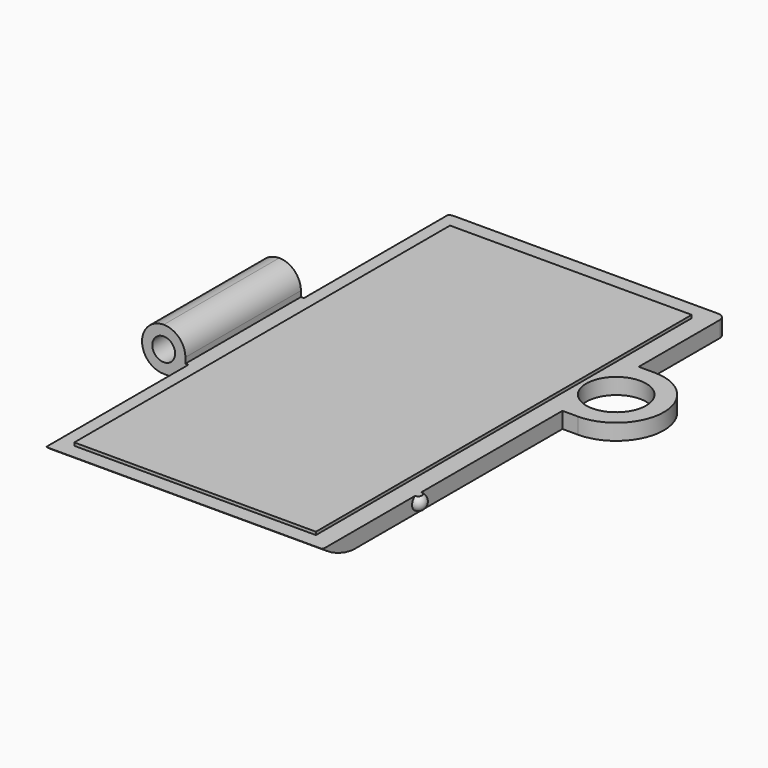
from build123d import *

# Parameters (mm, degrees)
F1_DEPTH  = 3.175
F2_R      = 5
F3_DEPTH  = 3.175
F4_W      = 7.239
F4_H      = 24.13
F5_DEPTH  = 7.239
F6_R      = 1.905
F7_DEPTH  = 25.4
F8_R      = 3.6195
F9_R      = 3.61949
F10_R     = 3.61949
F13_W     = 3.2799700804
F13_H     = 6.7503359169
F14_DEPTH = 0.5
F15_W     = 30.353
F15_H     = 2.675
F16_DEPTH = 0.5
F18_DEPTH = 46.236


# Not quite as in the source:
# - a fillet or chamfer is up to 0.001 mm smaller than in the source, because OpenCascade refuses the exact size


with BuildPart() as f1:
    # F0 (on Top) → F1 (new body)
    with BuildSketch(Plane.XY):
        with BuildLine():
            ThreePointArc((23.368, 41.148), (22.9960256121, 42.0460256121), (22.098, 42.418))
            Line((22.098, 42.418), (-22.098, 42.418))
            ThreePointArc((-22.098, 42.418), (-22.9960256121, 42.0460256121), (-23.368, 41.148))
            Line((-23.368, 41.148), (-23.368, -41.148))
            ThreePointArc((-23.368, -41.148), (-22.9960256121, -42.0460256121), (-22.098, -42.418))
            Line((-22.098, -42.418), (22.098, -42.418))
            ThreePointArc((22.098, -42.418), (22.9960256121, -42.0460256121), (23.368, -41.148))
            Line((23.368, -41.148), (23.368, 8.2812636))
            Line((23.368, 8.2812636), (23.368, 24.2070636))
            Line((23.368, 24.2070636), (23.368, 41.148))
        make_face()
        with BuildLine():
            Line((25.980898, 24.2070636), (23.368, 24.2070636))
            Line((23.368, 24.2070636), (23.368, 8.2812636))
            Line((23.368, 8.2812636), (25.980898, 8.2812636))
            ThreePointArc((25.980898, 8.2812636), (33.943798, 16.2441636), (25.980898, 24.2070636))
        make_face()
    extrude(amount=F1_DEPTH)

    # F2 (on face) → F3 (cut)
    with BuildSketch(Plane.XY.offset(3.175)):
        with Locations((25.980898, 16.2441636)):
            Circle(F2_R)
    extrude(amount=-F3_DEPTH, mode=Mode.SUBTRACT)

    # F4 (on face) → F5 (join)
    with BuildSketch(Plane(origin=(0, 0, 0), x_dir=(1, 0, 0), z_dir=(0, 0, -1))):
        with Locations((-26.9875, 0)):
            Rectangle(F4_W, F4_H)
    extrude(amount=-F5_DEPTH)

    # F6 (on face) → F7 (cut)
    with BuildSketch(Plane.XZ.offset(12.065)):
        with Locations((-26.9875, 3.6195)):
            Circle(F6_R)
    extrude(amount=-F7_DEPTH, mode=Mode.SUBTRACT)

    # F8
    f8_edges = [f1.edges().sort_by_distance(p)[0] for p in [
        (-30.607, 0, 7.239),
    ]]
    fillet(f8_edges, radius=F8_R)

    # F9 (radius 3.6195 in the source; OpenCascade refuses exactly that, so slightly less here)
    f9_edges = [f1.edges().sort_by_distance(p)[0] for p in [
        (-23.368, 0, 7.239),
    ]]
    fillet(f9_edges, radius=F9_R)

    # F10 (radius 3.6195 in the source; OpenCascade refuses exactly that, so slightly less here)
    f10_edges = [f1.edges().sort_by_distance(p)[0] for p in [
        (-30.607, 0, 0),
    ]]
    fillet(f10_edges, radius=F10_R)

    # F11 (on face) → F12 (revolve)
    with BuildSketch(Plane.YZ.offset(23.368)):
        with BuildLine():
            Line((-21.8558364, 2.8575), (-21.8558364, 0.3175))
            ThreePointArc((-21.8558364, 0.3175), (-20.5858364, 1.5875), (-21.8558364, 2.8575))
        make_face()
    revolve(axis=Axis((23.368, -21.8558364, 1.4411548618), (0, 0, 1)))

    # F13 (on face) → F14 (cut)
    with BuildSketch(Plane.XY.offset(3.175)):
        with BuildLine():
            Line((-23.368, -12.065), (-23.368, -42.418))
            Line((-23.368, -42.418), (23.368, -42.418))
            Line((23.368, -42.418), (23.368, -25.3541376442))
            Line((23.368, -25.3541376442), (23.368, -18.6038017273))
            Line((23.368, -18.6038017273), (23.368, 8.2812636))
            Line((23.368, 8.2812636), (25.980898, 8.2812636))
            ThreePointArc((25.980898, 8.2812636), (33.943798, 16.2441636), (25.980898, 24.2070636))
            Line((25.980898, 24.2070636), (23.368, 24.2070636))
            Line((23.368, 24.2070636), (23.368, 42.418))
            Line((23.368, 42.418), (-23.368, 42.418))
            Line((-23.368, 42.418), (-23.368, 12.065))
            Line((-23.368, 12.065), (-23.368, -12.065))
        make_face()
        Polygon((-20.193, 39.243), (20.193, 39.243), (20.193, 22.1750636), (20.193, 10.3132636), (20.193, -39.243), (-20.193, -39.243), (-20.193, -12.065), (-20.193, 12.065), align=None, mode=Mode.SUBTRACT)
        with Locations((25.0079850402, -21.9789696857)):
            Rectangle(F13_W, F13_H)
    extrude(amount=-F14_DEPTH, mode=Mode.SUBTRACT)

    # F15 (on face) → F16 (cut)
    with BuildSketch(Plane(origin=(-23.368, 0, 0), x_dir=(0, -1, 0), z_dir=(-1, 0, 0))):
        with Locations((-27.2415, 1.3375)):
            Rectangle(F15_W, F15_H)
        with Locations((27.2415, 1.3375)):
            Rectangle(F15_W, F15_H)
    extrude(amount=-F16_DEPTH, mode=Mode.SUBTRACT)

    # F17 (on face) → F18 (cut, through all)
    with BuildSketch(Plane(origin=(-22.868, 0, 0), x_dir=(0, -1, 0), z_dir=(-1, 0, 0))):
        with BuildLine():
            ThreePointArc((44.0055, 4.9726288032), (40.2838486613, 1.63965752), (35.5646422155, 0))
            Line((35.5646422155, 0), (44.0055, 0))
            Line((44.0055, 0), (44.0055, 4.9726288032))
        make_face()
    extrude(amount=-F18_DEPTH, mode=Mode.SUBTRACT)


solid = f1.part
